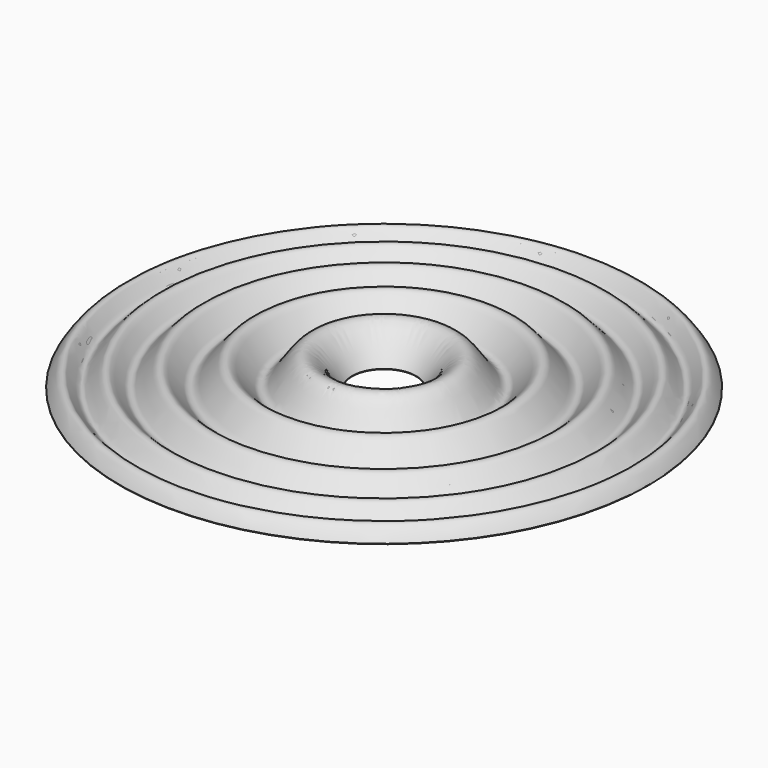
from build123d import *


with BuildPart() as f1:
    # F0 (on Front) → F1 (revolve)
    with BuildSketch(Plane.XZ):
        with BuildLine():
            Line((19.05, 0.254), (19.05, 0))
            add(Edge.make_bspline(
                [(19.05, 0), (19.8851835798, 1.1762377257), (40.7240775716, 35.917482442), (56.1852002036, -15.9989475478), (73.8010916579, 28.5019531694), (89.9252818373, -12.6173352435), (104.0894959727, 22.3365876708), (118.0541077279, -10.026283404), (129.4020541963, 17.996704012), (141.2217508471, -8.300957433), (149.1136098889, 14.9880755506), (156.9011944456, 0.802167557), (157.48, 0)],
                knots=[0, 0, 0, 0, 0.1213224661, 0.242346197, 0.3526052717, 0.4625190791, 0.5623463952, 0.6617795883, 0.7518299287, 0.8414403378, 0.9225743849, 1, 1, 1, 1], degree=3))
            Line((157.48, 0), (157.48, 0.254))
            add(Edge.make_bspline(
                [(19.05, 0.254), (19.7945829304, 1.6881054483), (40.766169356, 36.0516781984), (56.1750397608, -15.7160203667), (73.8037060447, 28.7484836229), (89.9246510286, -12.3614377588), (104.0896740484, 22.5897884294), (118.0540728767, -9.7709649323), (129.4020466206, 18.2459853097), (141.2217502728, -8.0299945859), (149.1136100382, 15.1864577427), (156.9011944456, 1.1707379802), (157.48, 0.254)],
                knots=[0, 0, 0, 0, 0.1213224149, 0.2423460946, 0.3526051227, 0.4625188837, 0.5623461576, 0.6617795115, 0.7518300335, 0.8414404049, 0.9225744176, 1, 1, 1, 1], degree=3))
        make_face()
    revolve(axis=Axis((0, 0, -2.7565898238), (0, 0, -1)))


solid = f1.part
